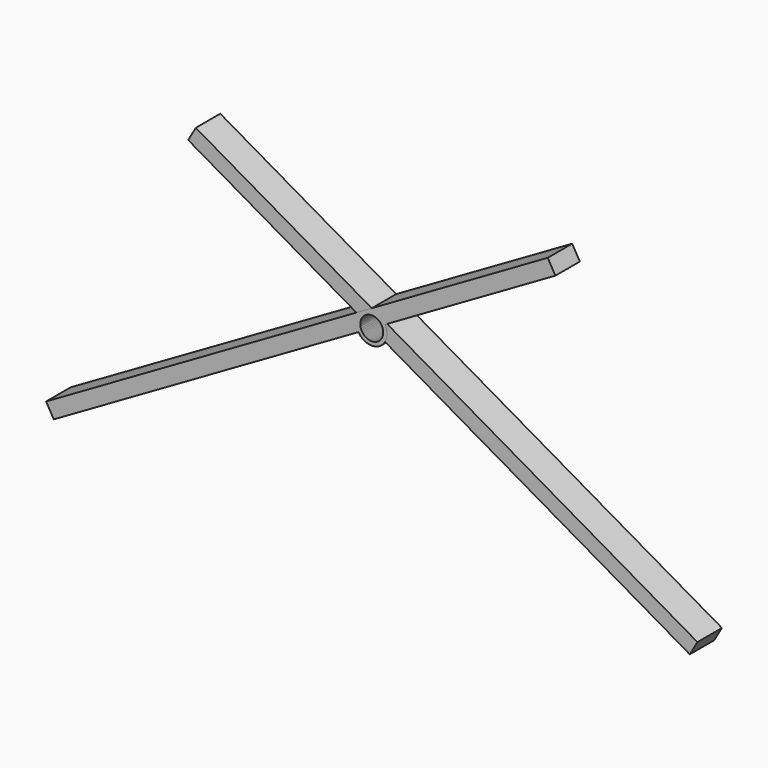
from build123d import *

# Parameters (mm, degrees)
F1_DEPTH = 12.7


with BuildPart() as f1:
    # F0 (on Front) → F1 (new body, symmetric)
    with BuildSketch(Plane.XZ):
        with BuildLine():
            Line((-152.4, 87.988181), (-10.998523, 6.35))
            ThreePointArc((-10.998523, 6.35), (-3.287002, 12.267258), (6.35, 10.998523))
            Line((6.35, 10.998523), (-146.05, 98.986704))
            Line((-146.05, 98.986704), (-152.4, 87.988181))
        make_face()
        with BuildLine():
            Line((8.248892, -4.7625), (10.998523, -6.35))
            ThreePointArc((10.998523, -6.35), (12.267258, -3.287002), (12.7, 0))
            ThreePointArc((12.7, 0), (10.998523, 6.35), (6.35, 10.998523))
            ThreePointArc((6.35, 10.998523), (-3.287002, 12.267258), (-10.998523, 6.35))
            Line((-10.998523, 6.35), (-8.248892, 4.7625))
            ThreePointArc((-8.248892, 4.7625), (2.465251, 9.200443), (9.525, 0))
            ThreePointArc((9.525, 0), (9.200443, -2.465251), (8.248892, -4.7625))
        make_face()
        with BuildLine():
            ThreePointArc((-10.998523, 6.35), (-6.35, -10.998523), (10.998523, -6.35))
            Line((10.998523, -6.35), (8.248892, -4.7625))
            ThreePointArc((8.248892, -4.7625), (-4.7625, -8.248892), (-8.248892, 4.7625))
            Line((-8.248892, 4.7625), (-10.998523, 6.35))
        make_face()
        with BuildLine():
            Line((10.998523, -6.35), (263.964543, -152.4))
            Line((263.964543, -152.4), (270.314543, -141.401477))
            Line((270.314543, -141.401477), (6.35, 10.998523))
            ThreePointArc((6.35, 10.998523), (10.998523, 6.35), (12.7, 0))
            ThreePointArc((12.7, 0), (12.267258, -3.287002), (10.998523, -6.35))
        make_face()
    extrude(amount=F1_DEPTH, both=True)


with BuildPart() as f2_1:
    # F2: instance of F1
    add(f1.part.mirror(Plane.YZ))


solid = Compound([f1.part, f2_1.part])
